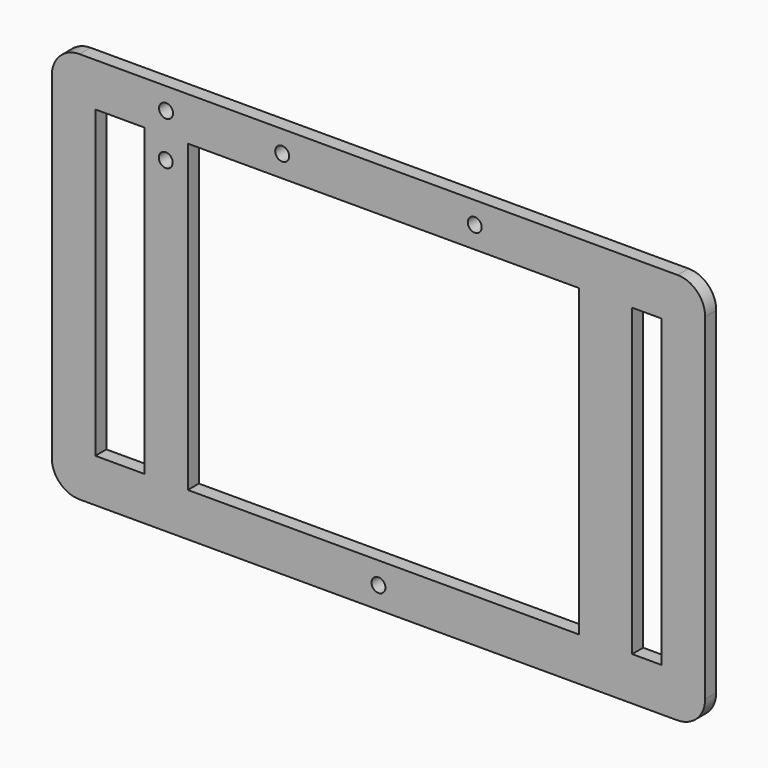
from build123d import *

# Parameters (mm, degrees)
F0_R     = 1.6
F0_W     = 11.2395305085
F0_H     = 70
F0_W_2   = 89.7604694915
F0_W_3   = 6.7604694915
F1_DEPTH = 3.175


# Not quite as in the source:
# - a length typed as a fraction of an inch, garbled in the dataset ("3 / 203.2 mm" for 3/8 in), is restored


with BuildPart() as f1:
    # F0 (on Front) → F1 (new body)
    with BuildSketch(Plane.XZ):
        with BuildLine():
            Line((21.2395305085, 0), (6.35, 0))
            ThreePointArc((6.35, 0), (1.8598719395, -1.8598719395), (0, -6.35))
            Line((0, -6.35), (0, -83.65))
            ThreePointArc((0, -83.65), (1.8598719395, -88.1401280605), (6.35, -90))
            Line((6.35, -90), (21.2395305085, -90))
            Line((21.2395305085, -90), (31.2395305085, -90))
            Line((31.2395305085, -90), (143.65, -90))
            ThreePointArc((143.65, -90), (148.1401280605, -88.1401280605), (150, -83.65))
            Line((150, -83.65), (150, -6.35))
            ThreePointArc((150, -6.35), (148.1401280605, -1.8598719395), (143.65, 0))
            Line((143.65, 0), (31.2395305085, 0))
            Line((31.2395305085, 0), (21.2395305085, 0))
        make_face()
        with Locations((75, -85)):
            Circle(F0_R, mode=Mode.SUBTRACT)
        with Locations((15.6197652543, -45)):
            Rectangle(F0_W, F0_H, mode=Mode.SUBTRACT)
        with Locations((26.162, -14.986)):
            Circle(F0_R, mode=Mode.SUBTRACT)
        with Locations((26.2395305085, -5)):
            Circle(F0_R, mode=Mode.SUBTRACT)
        with Locations((52.9, -5)):
            Circle(F0_R, mode=Mode.SUBTRACT)
        with Locations((76.1197652543, -45)):
            Rectangle(F0_W_2, F0_H, mode=Mode.SUBTRACT)
        with Locations((136.6197652543, -45)):
            Rectangle(F0_W_3, F0_H, mode=Mode.SUBTRACT)
        with Locations((97.1, -5)):
            Circle(F0_R, mode=Mode.SUBTRACT)
    extrude(amount=F1_DEPTH)


solid = f1.part
